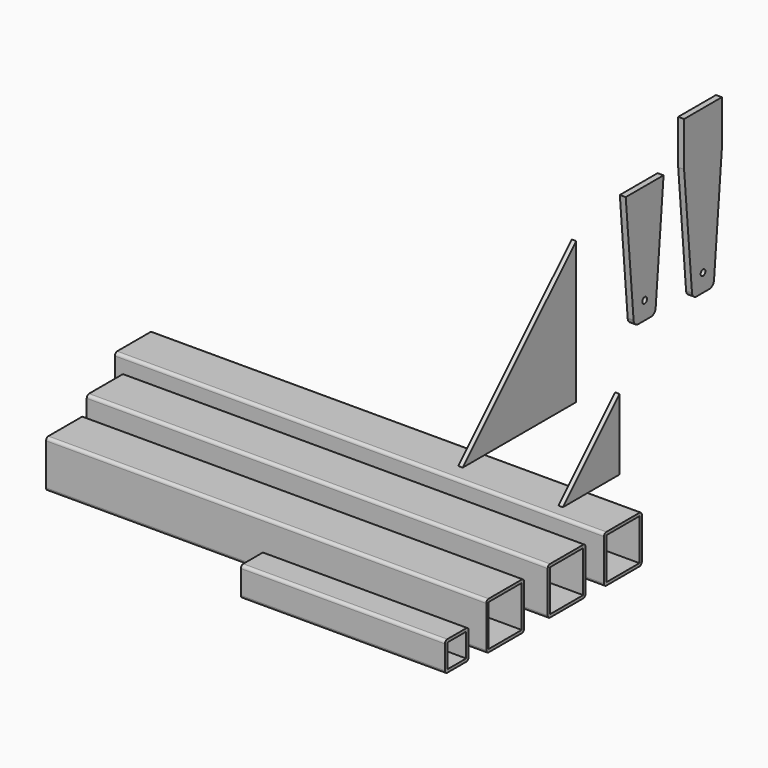
from build123d import *

# Parameters (mm, degrees)
F2_W      = 44.45
F2_H      = 44.45
F4_DEPTH  = 525.526
F0_W      = 44.45
F0_H      = 44.45
F5_DEPTH  = 495.3
F1_W      = 44.45
F1_H      = 44.45
F6_DEPTH  = 472.948
F3_W      = 25.4
F3_H      = 25.4
F9_DEPTH  = 219.202
F13_R     = 3.175
F15_DEPTH = 6.35
F18_R     = 3.175
F19_DEPTH = 6.35
F22_DEPTH = 4.7752
F25_DEPTH = 4.7752


# Not quite as in the source:
# - ends of sketch curves that miss each other by under 0.0002 mm in the source are joined


with BuildPart() as f4:
    # F2 (on Right) → F4 (new body)
    with BuildSketch(Plane.YZ):
        with BuildLine():
            ThreePointArc((73.8083965421, 73.8794356942), (72.8784605723, 76.1244997245), (70.6333965421, 77.0544356942))
            Line((70.6333965421, 77.0544356942), (26.1833965421, 77.0544356942))
            ThreePointArc((26.1833965421, 77.0544356942), (23.9383325118, 76.1244997245), (23.0083965421, 73.8794356942))
            Line((23.0083965421, 73.8794356942), (23.0083965421, 29.4294356942))
            ThreePointArc((23.0083965421, 29.4294356942), (23.9383325118, 27.184371664), (26.1833965421, 26.2544356942))
            Line((26.1833965421, 26.2544356942), (70.6333965421, 26.2544356942))
            ThreePointArc((70.6333965421, 26.2544356942), (72.8784605723, 27.184371664), (73.8083965421, 29.4294356942))
            Line((73.8083965421, 29.4294356942), (73.8083965421, 73.8794356942))
        make_face()
        with Locations((48.4083965421, 51.6544356942)):
            Rectangle(F2_W, F2_H, mode=Mode.SUBTRACT)
    extrude(amount=-F4_DEPTH)


with BuildPart() as f5:
    # F0 (on Right) → F5 (new body)
    with BuildSketch(Plane.YZ):
        with BuildLine():
            ThreePointArc((25.4, 22.225), (24.4700640303, 24.4700640303), (22.225, 25.4))
            Line((22.225, 25.4), (-22.225, 25.4))
            ThreePointArc((-22.225, 25.4), (-24.4700640303, 24.4700640303), (-25.4, 22.225))
            Line((-25.4, 22.225), (-25.4, -22.225))
            ThreePointArc((-25.4, -22.225), (-24.4700640303, -24.4700640303), (-22.225, -25.4))
            Line((-22.225, -25.4), (22.225, -25.4))
            ThreePointArc((22.225, -25.4), (24.4700640303, -24.4700640303), (25.4, -22.225))
            Line((25.4, -22.225), (25.4, 22.225))
        make_face()
        Rectangle(F0_W, F0_H, mode=Mode.SUBTRACT)
    extrude(amount=-F5_DEPTH)


with BuildPart() as f6:
    # F1 (on Right) → F6 (new body)
    with BuildSketch(Plane.YZ):
        with BuildLine():
            ThreePointArc((-58.2296081543, 45.6926692635), (-59.159544124, 47.9377332937), (-61.4046081543, 48.8676692635))
            Line((-61.4046081543, 48.8676692635), (-105.8546081543, 48.8676692635))
            ThreePointArc((-105.8546081543, 48.8676692635), (-108.0996721846, 47.9377332937), (-109.0296081543, 45.6926692635))
            Line((-109.0296081543, 45.6926692635), (-109.0296081543, 1.2426692635))
            ThreePointArc((-109.0296081543, 1.2426692635), (-108.0996721846, -1.0023947668), (-105.8546081543, -1.9323307365))
            Line((-105.8546081543, -1.9323307365), (-61.4046081543, -1.9323307365))
            ThreePointArc((-61.4046081543, -1.9323307365), (-59.159544124, -1.0023947668), (-58.2296081543, 1.2426692635))
            Line((-58.2296081543, 1.2426692635), (-58.2296081543, 45.6926692635))
        make_face()
        with Locations((-83.6296081543, 23.4676692635)):
            Rectangle(F1_W, F1_H, mode=Mode.SUBTRACT)
    extrude(amount=-F6_DEPTH)


with BuildPart() as f4_1:
    # F7: moved
    add(f4.part.moved(Location((0, 0, 54.67411))))


with BuildPart() as f6_1:
    # F8: moved
    add(f6.part.moved(Location((0, -96.26998, 0))))


with BuildPart() as f9:
    # F3 (on Right) → F9 (new body)
    with BuildSketch(Plane.YZ):
        with BuildLine():
            Line((-60.3392917745, -109.2081953526), (-34.9392917745, -109.2081953526))
            ThreePointArc((-34.9392917745, -109.2081953526), (-32.6942277442, -108.2782593828), (-31.7642917745, -106.0331953526))
            Line((-31.7642917745, -106.0331953526), (-31.7642917745, -80.6331953526))
            ThreePointArc((-31.7642917745, -80.6331953526), (-32.6942277442, -78.3881313223), (-34.9392917745, -77.4581953526))
            Line((-34.9392917745, -77.4581953526), (-60.3392917745, -77.4581953526))
            ThreePointArc((-60.3392917745, -77.4581953526), (-62.5843558047, -78.3881313223), (-63.5142917745, -80.6331953526))
            Line((-63.5142917745, -80.6331953526), (-63.5142917745, -106.0331953526))
            ThreePointArc((-63.5142917745, -106.0331953526), (-62.5843558047, -108.2782593828), (-60.3392917745, -109.2081953526))
        make_face()
        with Locations((-47.6392917745, -93.3331953526)):
            Rectangle(F3_W, F3_H, mode=Mode.SUBTRACT)
    extrude(amount=-F9_DEPTH)


with BuildPart() as f4_2:
    # F10: moved
    add(f4_1.part.moved(Location((0, 40.39893, -107.46899))))


with BuildPart() as f6_2:
    # F11: moved
    add(f6_1.part.moved(Location((0, 110.60677, -23.53336))))


with BuildPart() as f9_1:
    # F12: moved
    add(f9.part.moved(Location((0, -86.68119, 87.07341))))


with BuildPart() as f5_1:
    # F14: moved
    add(f5.part.moved(Location((0, 28.28909, -254.67151))))


with BuildPart() as f15:
    # F13 (on Right) → F15 (new body)
    with BuildSketch(Plane.YZ):
        with BuildLine():
            Line((14.7960588, -81.5159406), (25.4, 39.6875))
            Line((25.4, 39.6875), (25.4, 87.3125))
            Line((25.4, 87.3125), (-25.4, 87.3125))
            Line((-25.4, 87.3125), (-25.4, 39.6875))
            Line((-25.4, 39.6875), (-14.7960842, -81.5159406))
            ThreePointArc((-14.7960842, -81.5159406), (-12.7602370841, -85.6442113951), (-8.4702396, -87.3125))
            Line((-8.4702396, -87.3125), (8.4702396, -87.3125))
            ThreePointArc((8.4702396, -87.3125), (12.760236268, -85.6442121429), (14.7960588, -81.5159406))
        make_face()
        with Locations((0, -68.2625)):
            Circle(F13_R, mode=Mode.SUBTRACT)
    extrude(amount=F15_DEPTH)


with BuildPart() as f15_1:
    # F16: moved
    add(f15.part.moved(Location((0, 203.53773, 36.31291))))


with BuildPart() as f9_2:
    # F17: moved
    add(f9_1.part.moved(Location((0, 15.0572, -253.99659))))


with BuildPart() as f6_3:
    # F17: moved
    add(f6_2.part.moved(Location((0, 15.0572, -253.99659))))


with BuildPart() as f4_3:
    # F17: moved
    add(f4_2.part.moved(Location((0, 15.0572, -253.99659))))


with BuildPart() as f19:
    # F18 (on Right) → F19 (new body)
    with BuildSketch(Plane.YZ):
        with BuildLine():
            Line((14.7960842, -57.7034406), (25.4, 63.5))
            Line((25.4, 63.5), (-25.4, 63.5))
            Line((-25.4, 63.5), (-14.842363, -57.1741554))
            Line((-14.842363, -57.1741554), (-14.7960588, -57.7034406))
            ThreePointArc((-14.7960588, -57.7034406), (-12.7602116841, -61.8317113951), (-8.4702142, -63.5))
            Line((-8.4702142, -63.5), (8.4702396, -63.5))
            ThreePointArc((8.4702396, -63.5), (12.7602370841, -61.8317113951), (14.7960842, -57.7034406))
        make_face()
        with Locations((0, -44.45)):
            Circle(F18_R, mode=Mode.SUBTRACT)
    extrude(amount=F19_DEPTH)


with BuildPart() as f19_1:
    # F20: moved
    add(f19.part.moved(Location((0, 125.14704, 18.10973))))


with BuildPart() as f22:
    # F21 (on Right) → F22 (new body)
    with BuildSketch(Plane.YZ):
        Polygon((16.7840082307, 37.6099455118), (-59.4159917693, -38.5900544882), (16.7840082307, -38.5900544882), align=None)
    extrude(amount=F22_DEPTH)


with BuildPart() as f22_1:
    # F23: moved
    add(f22.part.moved(Location((0, 76.67682, -140.10945))))


with BuildPart() as f25:
    # F24 (on Right) → F25 (new body)
    with BuildSketch(Plane.YZ):
        Polygon((35.1358502615, -86.559140113), (35.1358502615, 65.840859887), (-117.2641497385, -86.559140113), align=None)
    extrude(amount=F25_DEPTH)


solid = Compound([f5_1.part, f15_1.part, f9_2.part, f6_3.part, f4_3.part, f19_1.part, f22_1.part, f25.part])
